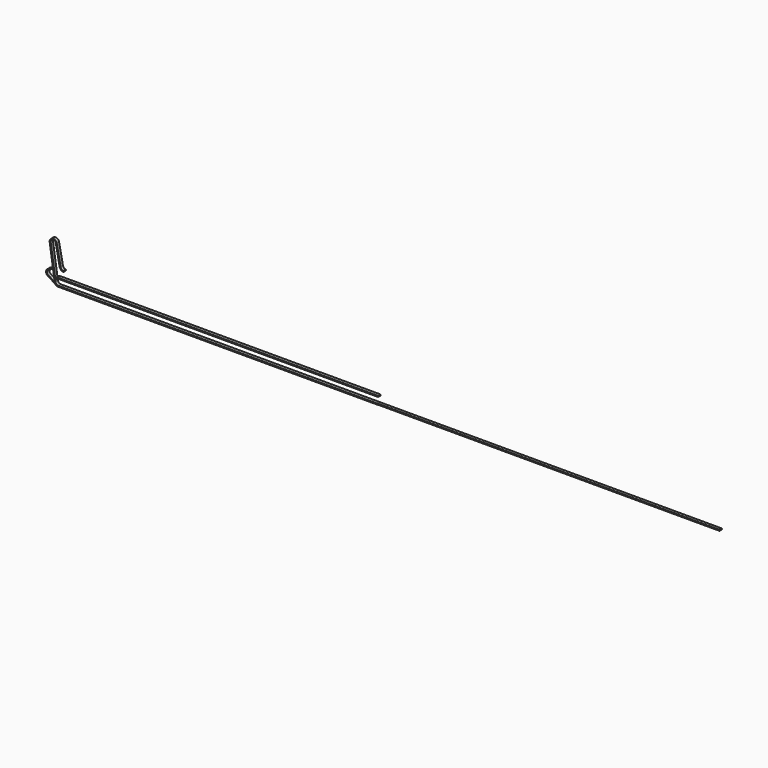
from build123d import *

# Parameters (mm, degrees)
F1_DEPTH = 6
F2_DEPTH = 6
F3_DEPTH = 1124.746
F4_DEPTH = 900
F5_DEPTH = 6
F6_DEPTH = 1138.825
F7_DEPTH = 6.5
F8_DEPTH = 650
F9_DEPTH = 445.0137512445


with BuildPart() as f1:
    # F0 (on Front) → F1 (new body)
    with BuildSketch(Plane.XZ):
        with BuildLine():
            ThreePointArc((-95.136328143, 4.9075490426), (-95.044474725, 7.7986213794), (-93.9426587116, 10.4730816576))
            Line((-93.9426587116, 10.4730816576), (-102.4278166884, 67.4824899201))
            Line((-102.4278166884, 67.4824899201), (-103.1668359845, 72.4477543118))
            ThreePointArc((-103.1668359845, 72.4477543118), (-98.8281492163, 78.4504101753), (-92.7249162558, 74.2543849469))
            Line((-92.7249162558, 74.2543849469), (-91.7527631347, 69.3294566927))
            Line((-91.7527631347, 69.3294566927), (-84.8212434204, 34.214373949))
            ThreePointArc((-84.8212434204, 34.214373949), (-82.0177400253, 29.5253698171), (-76.8745829701, 27.683))
            Line((-76.8745829701, 27.683), (-76.8745829701, 29.683))
            ThreePointArc((-76.8745829701, 29.683), (-80.747824703, 31.0704636894), (-82.8591050376, 34.6016890233))
            Line((-82.8591050376, 34.6016890233), (-83.891138014, 39.8299686578))
            Line((-83.891138014, 39.8299686578), (-90.762777873, 74.6417000212))
            ThreePointArc((-90.762777873, 74.6417000212), (-99.169117611, 80.4211309961), (-105.1450446691, 72.1533219767))
            Line((-105.1450446691, 72.1533219767), (-95.136328143, 4.9075490426))
        make_face()
        with BuildLine():
            ThreePointArc((-90.3982102295, 0.9528294601), (-92.2402107186, 2.7772973742), (-93.1581194583, 5.2019813778))
            Line((-93.1581194583, 5.2019813778), (-93.9426587116, 10.4730816576))
            ThreePointArc((-93.9426587116, 10.4730816576), (-95.044474725, 7.7986213794), (-95.136328143, 4.9075490426))
            ThreePointArc((-95.136328143, 4.9075490426), (-95.0346023946, 4.3559837432), (-94.8949514237, 3.8127802695))
            Line((-94.8949514237, 3.8127802695), (-90.3982102295, 0.9528294601))
        make_face()
        with BuildLine():
            Line((117.8616657853, 0), (-81.7954179324, 0))
            ThreePointArc((-81.7954179324, 0), (-84.278533076, -1.4835347959), (-87.1245829701, -2))
            Line((-87.1245829701, -2), (117.8616657853, -2))
            Line((117.8616657853, -2), (117.8616657853, 0))
        make_face()
        with BuildLine():
            Line((-81.7954179324, 0), (-87.1245829701, 0))
            ThreePointArc((-87.1245829701, 0), (-88.8293204436, 0.2430494157), (-90.3982102295, 0.9528294601))
            Line((-90.3982102295, 0.9528294601), (-94.8949514237, 3.8127802695))
            ThreePointArc((-94.8949514237, 3.8127802695), (-93.5958568063, 1.2283868239), (-91.4715306424, -0.7347674382))
            ThreePointArc((-91.4715306424, -0.7347674382), (-89.3882507627, -1.6772622513), (-87.1245829701, -2))
            ThreePointArc((-87.1245829701, -2), (-84.278533076, -1.4835347959), (-81.7954179324, 0))
        make_face()
    extrude(amount=F1_DEPTH)


with BuildPart() as f2:
    # F0 (on Front) → F2 (new body)
    with BuildSketch(Plane.XZ):
        with BuildLine():
            Line((-81.7954179324, 0), (-87.1245829701, 0))
            ThreePointArc((-87.1245829701, 0), (-88.8293204436, 0.2430494157), (-90.3982102295, 0.9528294601))
            Line((-90.3982102295, 0.9528294601), (-94.8949514237, 3.8127802695))
            ThreePointArc((-94.8949514237, 3.8127802695), (-93.5958568063, 1.2283868239), (-91.4715306424, -0.7347674382))
            ThreePointArc((-91.4715306424, -0.7347674382), (-89.3882507627, -1.6772622513), (-87.1245829701, -2))
            ThreePointArc((-87.1245829701, -2), (-84.278533076, -1.4835347959), (-81.7954179324, 0))
        make_face()
        with BuildLine():
            ThreePointArc((-93.1581194583, 5.2019813778), (-91.7445350043, 10.0832202051), (-87.1245829701, 12.2))
            Line((-87.1245829701, 12.2), (-87.1245829701, 14.2))
            ThreePointArc((-87.1245829701, 14.2), (-91.0096851936, 13.2074595119), (-93.9426587116, 10.4730816576))
            Line((-93.9426587116, 10.4730816576), (-93.1581194583, 5.2019813778))
        make_face()
        with BuildLine():
            ThreePointArc((-90.3982102295, 0.9528294601), (-92.2402107186, 2.7772973742), (-93.1581194583, 5.2019813778))
            Line((-93.1581194583, 5.2019813778), (-93.9426587116, 10.4730816576))
            ThreePointArc((-93.9426587116, 10.4730816576), (-95.044474725, 7.7986213794), (-95.136328143, 4.9075490426))
            ThreePointArc((-95.136328143, 4.9075490426), (-95.0346023946, 4.3559837432), (-94.8949514237, 3.8127802695))
            Line((-94.8949514237, 3.8127802695), (-90.3982102295, 0.9528294601))
        make_face()
        with BuildLine():
            Line((117.8616657853, 0), (-81.7954179324, 0))
            ThreePointArc((-81.7954179324, 0), (-84.278533076, -1.4835347959), (-87.1245829701, -2))
            Line((-87.1245829701, -2), (117.8616657853, -2))
            Line((117.8616657853, -2), (117.8616657853, 0))
        make_face()
    extrude(amount=F2_DEPTH)


with BuildPart() as f3:
    # F3 (new): a face of the model
    f3_faces = [f1.part.faces().sort_by_distance(p)[0] for p in [
        (117.8616657853, -3, -1),
    ]]
    extrude(f3_faces, amount=F3_DEPTH)


with BuildPart() as f4:
    # F4 (new): a face of the model
    f4_faces = [f1.part.faces().sort_by_distance(p)[0] for p in [
        (117.8616657853, -3, -1),
    ]]
    extrude(f4_faces, amount=F4_DEPTH)


with BuildPart() as f5:
    # F0 (on Front) → F5 (new body)
    with BuildSketch(Plane.XZ):
        with BuildLine():
            ThreePointArc((-109.0422024773, 10.4402713211), (-106.4841760595, 9.4277265368), (-103.7330474672, 9.433855364))
            Line((-103.7330474672, 9.433855364), (-107.9688820644, 12.1278682194))
            ThreePointArc((-107.9688820644, 12.1278682194), (-110.2134088876, 18.0811653458), (-105.1245829701, 21.9))
            Line((-105.1245829701, 21.9), (-105.049590473, 23.8996147929))
            ThreePointArc((-105.049590473, 23.8996147929), (-112.123149056, 18.6760714685), (-109.0422024773, 10.4402713211))
        make_face()
        with BuildLine():
            ThreePointArc((-91.4715306424, -0.7347674382), (-93.5958568063, 1.2283868239), (-94.8949514237, 3.8127802695))
            Line((-94.8949514237, 3.8127802695), (-103.7330474672, 9.433855364))
            ThreePointArc((-103.7330474672, 9.433855364), (-106.4841760595, 9.4277265368), (-109.0422024773, 10.4402713211))
            Line((-109.0422024773, 10.4402713211), (-91.4715306424, -0.7347674382))
        make_face()
        with BuildLine():
            Line((-81.7954179324, 0), (-87.1245829701, 0))
            ThreePointArc((-87.1245829701, 0), (-88.8293204436, 0.2430494157), (-90.3982102295, 0.9528294601))
            Line((-90.3982102295, 0.9528294601), (-94.8949514237, 3.8127802695))
            ThreePointArc((-94.8949514237, 3.8127802695), (-93.5958568063, 1.2283868239), (-91.4715306424, -0.7347674382))
            ThreePointArc((-91.4715306424, -0.7347674382), (-89.3882507627, -1.6772622513), (-87.1245829701, -2))
            ThreePointArc((-87.1245829701, -2), (-84.278533076, -1.4835347959), (-81.7954179324, 0))
        make_face()
        with BuildLine():
            Line((117.8616657853, 0), (-81.7954179324, 0))
            ThreePointArc((-81.7954179324, 0), (-84.278533076, -1.4835347959), (-87.1245829701, -2))
            Line((-87.1245829701, -2), (117.8616657853, -2))
            Line((117.8616657853, -2), (117.8616657853, 0))
        make_face()
    extrude(amount=F5_DEPTH)


with BuildPart() as f6:
    # F6 (new): a face of the model
    f6_faces = [f5.part.faces().sort_by_distance(p)[0] for p in [
        (117.8616657853, -3, -1),
    ]]
    extrude(f6_faces, amount=F6_DEPTH)


with BuildPart() as f7:
    # F0 (on Front) → F7 (new body)
    with BuildSketch(Plane.XZ):
        with BuildLine():
            ThreePointArc((-93.1581194583, 5.2019813778), (-91.7445350043, 10.0832202051), (-87.1245829701, 12.2))
            Line((-87.1245829701, 12.2), (-87.1245829701, 14.2))
            ThreePointArc((-87.1245829701, 14.2), (-91.0096851936, 13.2074595119), (-93.9426587116, 10.4730816576))
            Line((-93.9426587116, 10.4730816576), (-93.1581194583, 5.2019813778))
        make_face()
        with BuildLine():
            ThreePointArc((-90.3982102295, 0.9528294601), (-92.2402107186, 2.7772973742), (-93.1581194583, 5.2019813778))
            Line((-93.1581194583, 5.2019813778), (-93.9426587116, 10.4730816576))
            ThreePointArc((-93.9426587116, 10.4730816576), (-95.044474725, 7.7986213794), (-95.136328143, 4.9075490426))
            ThreePointArc((-95.136328143, 4.9075490426), (-95.0346023946, 4.3559837432), (-94.8949514237, 3.8127802695))
            Line((-94.8949514237, 3.8127802695), (-90.3982102295, 0.9528294601))
        make_face()
        with BuildLine():
            Line((-81.7954179324, 0), (-87.1245829701, 0))
            ThreePointArc((-87.1245829701, 0), (-88.8293204436, 0.2430494157), (-90.3982102295, 0.9528294601))
            Line((-90.3982102295, 0.9528294601), (-94.8949514237, 3.8127802695))
            ThreePointArc((-94.8949514237, 3.8127802695), (-93.5958568063, 1.2283868239), (-91.4715306424, -0.7347674382))
            ThreePointArc((-91.4715306424, -0.7347674382), (-89.3882507627, -1.6772622513), (-87.1245829701, -2))
            ThreePointArc((-87.1245829701, -2), (-84.278533076, -1.4835347959), (-81.7954179324, 0))
        make_face()
        with BuildLine():
            Line((117.8616657853, 0), (-81.7954179324, 0))
            ThreePointArc((-81.7954179324, 0), (-84.278533076, -1.4835347959), (-87.1245829701, -2))
            Line((-87.1245829701, -2), (117.8616657853, -2))
            Line((117.8616657853, -2), (117.8616657853, 0))
        make_face()
    extrude(amount=F7_DEPTH)

    # F8 (add): a face of the model
    f8_faces = [f7.faces().sort_by_distance(p)[0] for p in [
        (-87.1245829701, -3.25, 13.2),
    ]]
    extrude(f8_faces, amount=F8_DEPTH)

    # F9 (add, through all): a face of the model
    f9_faces = [f7.faces().sort_by_distance(p)[0] for p in [
        (117.8616657853, -3.25, -1),
    ]]
    extrude(f9_faces, amount=F9_DEPTH)


solid = Compound([f1.part, f2.part, f3.part, f4.part, f5.part, f6.part, f7.part])
